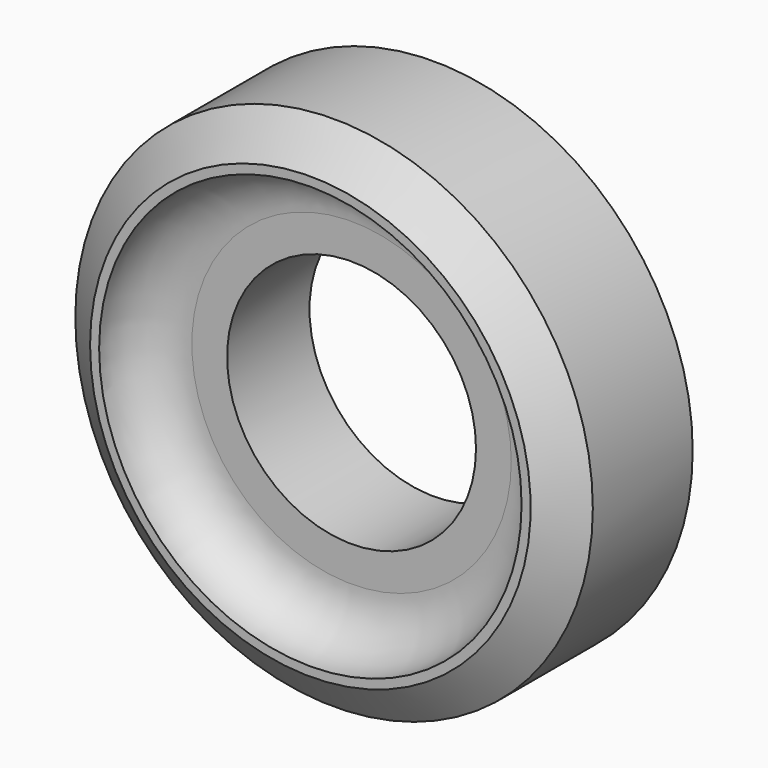
from build123d import *

# Parameters (mm, degrees)
F0_R     = 30.15
F1_DEPTH = 18
F2_R     = 24.61
F3_DEPTH = 6
F4_R     = 5.99999
F5_R     = 14.5
F6_DEPTH = 25


# Not quite as in the source:
# - a fillet or chamfer is up to 0.001 mm smaller than in the source, because OpenCascade refuses the exact size


with BuildPart() as f1:
    # F0 (on Front) → F1 (new body)
    with BuildSketch(Plane.XZ):
        Circle(F0_R)
    extrude(amount=F1_DEPTH)

    # F2 (on face) → F3 (cut)
    with BuildSketch(Plane.XZ.offset(18)):
        Circle(F2_R)
    extrude(amount=-F3_DEPTH, mode=Mode.SUBTRACT)

    # F4 (radius 6 in the source; OpenCascade refuses exactly that, so slightly less here)
    f4_edges = [f1.edges().sort_by_distance(p)[0] for p in [
        (-24.61, -12, 0),
    ]]
    fillet(f4_edges, radius=F4_R)

    # F5 (on face) → F6 (cut)
    with BuildSketch(Plane.XZ.offset(12)):
        Circle(F5_R)
    extrude(amount=-F6_DEPTH, mode=Mode.SUBTRACT)

    # F7 (on Top) → F8 (revolve, cut)
    with BuildSketch(Plane.XY):
        Polygon((-30.15, -18), (-25.6668464834, -18), (-30.15, -14.5470285541), align=None)
    revolve(axis=Axis((0, -2.2485724185, 0), (0, -1, 0)), mode=Mode.SUBTRACT)


solid = f1.part
